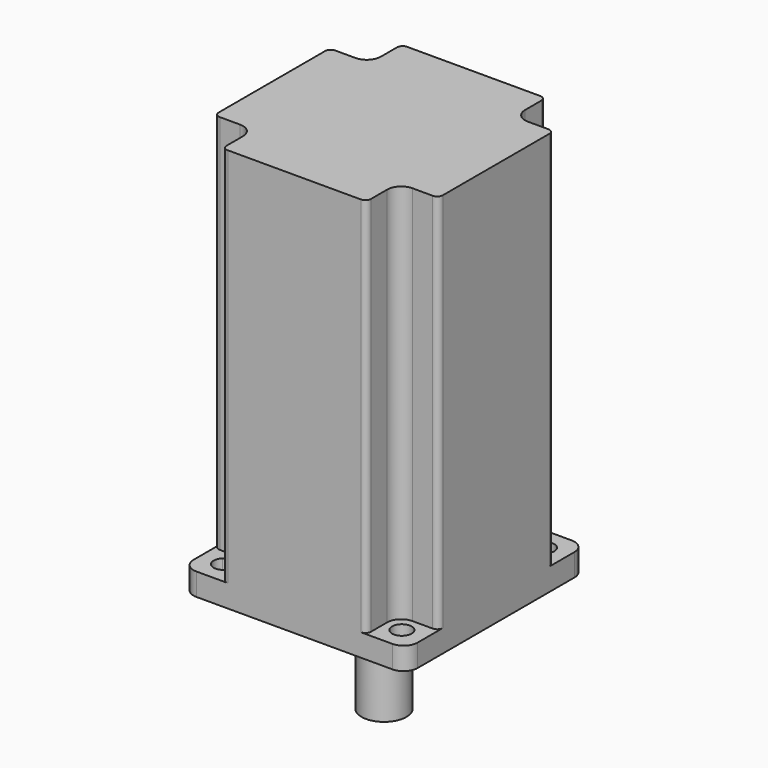
from build123d import *

# Parameters (mm, degrees)
F1_DEPTH = 8
F2_R     = 35
F3_DEPTH = 3
F4_R     = 8
F5_DEPTH = 37
F7_DEPTH = 136


# Not quite as in the source:
# - a feature names something its author has since deleted; it is built from what else it names


with BuildPart() as f1:
    # F0 (on Top) → F1 (new body)
    with BuildSketch(Plane.XY):
        with BuildLine():
            Line((-20.6155281281, 40), (-35, 40))
            ThreePointArc((-35, 40), (-38.5355339059, 38.5355339059), (-40, 35))
            Line((-40, 35), (-40, 20.6155281281))
            ThreePointArc((-40, 20.6155281281), (-37.348673038, 25.1013271024), (-34.1965616575, 29.25055847))
            ThreePointArc((-34.1965616575, 29.25055847), (-34.2946788875, 34.2946788875), (-29.25055847, 34.1965616575))
            ThreePointArc((-29.25055847, 34.1965616575), (-25.1013271024, 37.348673038), (-20.6155281281, 40))
        make_face()
        with BuildLine():
            ThreePointArc((-34.1965616575, 29.25055847), (-37.348673038, 25.1013271024), (-40, 20.6155281281))
            Line((-40, 20.6155281281), (-40, -20.6155281281))
            ThreePointArc((-40, -20.6155281281), (-37.348673038, -25.1013271024), (-34.1965616575, -29.25055847))
            ThreePointArc((-34.1965616575, -29.25055847), (-33.0960568151, -28.5607897045), (-31.8198051534, -28.3198051534))
            Line((-31.8198051534, -28.3198051534), (-31.8198051534, 28.3198051534))
            ThreePointArc((-31.8198051534, 28.3198051534), (-33.0960568151, 28.5607897045), (-34.1965616575, 29.25055847))
        make_face()
        with BuildLine():
            Line((28.3198051534, 31.8198051534), (-28.3198051534, 31.8198051534))
            ThreePointArc((-28.3198051534, 31.8198051534), (-29.3449314192, 29.3449314192), (-31.8198051534, 28.3198051534))
            Line((-31.8198051534, 28.3198051534), (-31.8198051534, -28.3198051534))
            ThreePointArc((-31.8198051534, -28.3198051534), (-29.3449314192, -29.3449314192), (-28.3198051534, -31.8198051534))
            ThreePointArc((-28.3198051534, -31.8198051534), (-28.5607897045, -33.0960568151), (-29.25055847, -34.1965616575))
            ThreePointArc((-29.25055847, -34.1965616575), (-25.1013271024, -37.348673038), (-20.6155281281, -40))
            Line((-20.6155281281, -40), (20.6155281281, -40))
            ThreePointArc((20.6155281281, -40), (25.1013271024, -37.348673038), (29.25055847, -34.1965616575))
            ThreePointArc((29.25055847, -34.1965616575), (29.3449314192, -29.3449314192), (34.1965616575, -29.25055847))
            ThreePointArc((34.1965616575, -29.25055847), (37.348673038, -25.1013271024), (40, -20.6155281281))
            Line((40, -20.6155281281), (40, 20.6155281281))
            ThreePointArc((40, 20.6155281281), (37.348673038, 25.1013271024), (34.1965616575, 29.25055847))
            ThreePointArc((34.1965616575, 29.25055847), (30.417779434, 28.612887025), (28.3198051534, 31.8198051534))
        make_face()
        with BuildLine():
            Line((20.6155281281, 40), (-20.6155281281, 40))
            ThreePointArc((-20.6155281281, 40), (-25.1013271024, 37.348673038), (-29.25055847, 34.1965616575))
            ThreePointArc((-29.25055847, 34.1965616575), (-28.5607897045, 33.0960568151), (-28.3198051534, 31.8198051534))
            Line((-28.3198051534, 31.8198051534), (28.3198051534, 31.8198051534))
            ThreePointArc((28.3198051534, 31.8198051534), (28.5607897045, 33.0960568151), (29.25055847, 34.1965616575))
            ThreePointArc((29.25055847, 34.1965616575), (25.1013271024, 37.348673038), (20.6155281281, 40))
        make_face()
        with BuildLine():
            Line((35, 40), (20.6155281281, 40))
            ThreePointArc((20.6155281281, 40), (25.1013271024, 37.348673038), (29.25055847, 34.1965616575))
            ThreePointArc((29.25055847, 34.1965616575), (33.0960568151, 35.0788206023), (35.3198051534, 31.8198051534))
            ThreePointArc((35.3198051534, 31.8198051534), (35.0267232818, 30.417779434), (34.1965616575, 29.25055847))
            ThreePointArc((34.1965616575, 29.25055847), (37.348673038, 25.1013271024), (40, 20.6155281281))
            Line((40, 20.6155281281), (40, 35))
            ThreePointArc((40, 35), (38.5355339059, 38.5355339059), (35, 40))
        make_face()
        with BuildLine():
            ThreePointArc((-34.1965616575, -29.25055847), (-37.348673038, -25.1013271024), (-40, -20.6155281281))
            Line((-40, -20.6155281281), (-40, -35))
            ThreePointArc((-40, -35), (-38.5355339059, -38.5355339059), (-35, -40))
            Line((-35, -40), (-20.6155281281, -40))
            ThreePointArc((-20.6155281281, -40), (-25.1013271024, -37.348673038), (-29.25055847, -34.1965616575))
            ThreePointArc((-29.25055847, -34.1965616575), (-34.2946788875, -34.2946788875), (-34.1965616575, -29.25055847))
        make_face()
        with BuildLine():
            Line((40, -35), (40, -20.6155281281))
            ThreePointArc((40, -20.6155281281), (37.348673038, -25.1013271024), (34.1965616575, -29.25055847))
            ThreePointArc((34.1965616575, -29.25055847), (35.0267232818, -30.417779434), (35.3198051534, -31.8198051534))
            ThreePointArc((35.3198051534, -31.8198051534), (33.0960568151, -35.0788206023), (29.25055847, -34.1965616575))
            ThreePointArc((29.25055847, -34.1965616575), (25.1013271024, -37.348673038), (20.6155281281, -40))
            Line((20.6155281281, -40), (35, -40))
            ThreePointArc((35, -40), (38.5355339059, -38.5355339059), (40, -35))
        make_face()
    extrude(amount=F1_DEPTH)

    # F2 (on face) → F3 (join)
    with BuildSketch(Plane(origin=(0, 0, 0), x_dir=(1, 0, 0), z_dir=(0, 0, -1))):
        Circle(F2_R)
    extrude(amount=F3_DEPTH)

    # F4 (on face) → F5 (join)
    with BuildSketch(Plane(origin=(0, 0, -3), x_dir=(1, 0, 0), z_dir=(0, 0, -1))):
        Circle(F4_R)
    extrude(amount=F5_DEPTH)

    # F6 (on face) → F7 (join)
    with BuildSketch(Plane.XY.offset(8)):
        with BuildLine():
            Line((-30.75, 25.75), (-38, 25.75))
            ThreePointArc((-38, 25.75), (-39.4142135624, 25.1642135624), (-40, 23.75))
            Line((-40, 23.75), (-40, -23.75))
            ThreePointArc((-40, -23.75), (-39.4142135624, -25.1642135624), (-38, -25.75))
            Line((-38, -25.75), (-30.75, -25.75))
            ThreePointArc((-30.75, -25.75), (-27.2144660941, -27.2144660941), (-25.75, -30.75))
            Line((-25.75, -30.75), (-25.75, -38))
            ThreePointArc((-25.75, -38), (-25.1642135624, -39.4142135624), (-23.75, -40))
            Line((-23.75, -40), (23.75, -40))
            ThreePointArc((23.75, -40), (25.1642135624, -39.4142135624), (25.75, -38))
            Line((25.75, -38), (25.75, -30.75))
            ThreePointArc((25.75, -30.75), (27.2144660941, -27.2144660941), (30.75, -25.75))
            Line((30.75, -25.75), (38, -25.75))
            ThreePointArc((38, -25.75), (39.4142135624, -25.1642135624), (40, -23.75))
            Line((40, -23.75), (40, 23.75))
            ThreePointArc((40, 23.75), (39.4142135624, 25.1642135624), (38, 25.75))
            Line((38, 25.75), (30.75, 25.75))
            ThreePointArc((30.75, 25.75), (27.2144660941, 27.2144660941), (25.75, 30.75))
            Line((25.75, 30.75), (25.75, 38))
            ThreePointArc((25.75, 38), (25.1642135624, 39.4142135624), (23.75, 40))
            Line((23.75, 40), (-23.75, 40))
            ThreePointArc((-23.75, 40), (-25.1642135624, 39.4142135624), (-25.75, 38))
            Line((-25.75, 38), (-25.75, 30.75))
            ThreePointArc((-25.75, 30.75), (-27.2144660941, 27.2144660941), (-30.75, 25.75))
        make_face()
    extrude(amount=F7_DEPTH)


solid = f1.part
